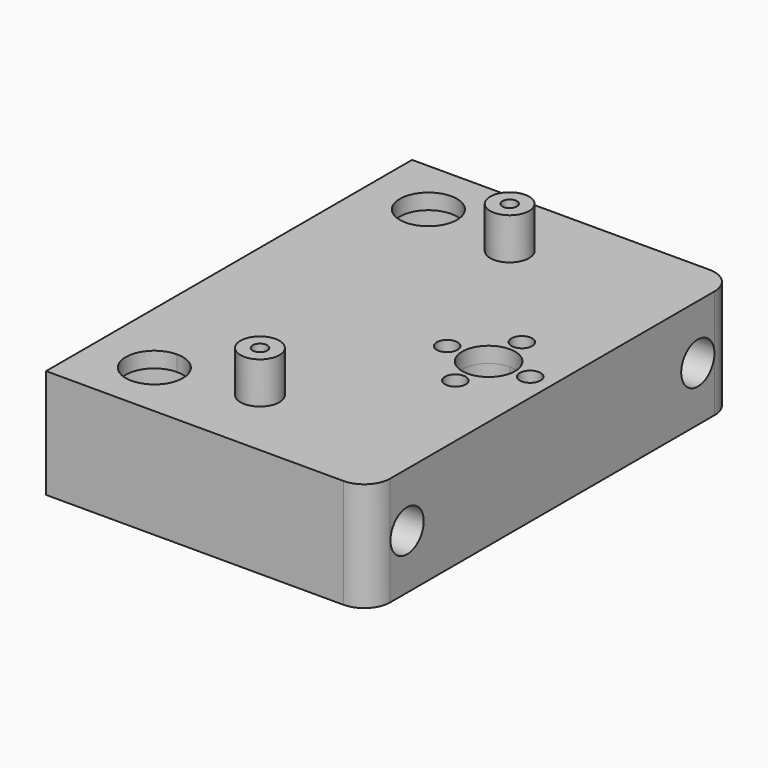
from build123d import *

# Parameters (mm, degrees)
F1_DEPTH  = 2
F2_R      = 9.75
F2_R_2    = 11.25
F2_R_3    = 2
F3_DEPTH  = 16
F4_R      = 9.75
F4_R_2    = 2
F4_R_3    = 5.1
F5_DEPTH  = 3
F7_DEPTH  = 40
F6_R      = 4
F8_DEPTH  = 35
F9_R      = 3.75
F9_R_2    = 1.4
F10_DEPTH = 8


# Not quite as in the source:
# - after a boolean that leaves OpenCascade's solid faulty, fix() repairs it
# - a feature names something its author has since deleted; it is built from what else it names


with BuildPart() as f1:
    # F0 (on Top) → F1 (new body)
    with BuildSketch(Plane.XY):
        with BuildLine():
            Line((50.2909459174, -23.5600714934), (50.2909459174, 23.5599285066))
            Line((50.2909459174, 23.5599285066), (50.2909459174, 39.0599285066))
            ThreePointArc((50.2909459174, 39.0599285066), (48.8264798233, 42.5954624125), (45.2909459174, 44.0599285066))
            Line((45.2909459174, 44.0599285066), (-12, 44.0599285066))
            Line((-12, 44.0599285066), (-12, 0))
            Line((-12, 0), (-12, -44.0599285066))
            Line((-12, -44.0599285066), (45.2909459174, -44.0599285066))
            ThreePointArc((45.2909459174, -44.0599285066), (48.8264798233, -42.5954624125), (50.2909459174, -39.0599285066))
            Line((50.2909459174, -39.0599285066), (50.2909459174, -23.5600714934))
        make_face()
        with BuildLine():
            ThreePointArc((9.75, -33), (-6.8942911166, -39.8942911166), (0, -23.25))
            ThreePointArc((0, -23.25), (6.8942911166, -26.1057088834), (9.75, -33))
        make_face(mode=Mode.SUBTRACT)
        with BuildLine():
            ThreePointArc((9.75, 33), (6.8942911166, 26.1057088834), (0, 23.25))
            ThreePointArc((0, 23.25), (-6.8942911166, 39.8942911166), (9.75, 33))
        make_face(mode=Mode.SUBTRACT)
        with BuildLine():
            ThreePointArc((26.75, 0), (38, 11.25), (49.25, 0))
            ThreePointArc((49.25, 0), (38, -11.25), (26.75, 0))
        make_face(mode=Mode.SUBTRACT)
    extrude(amount=F1_DEPTH)

    # F2 (on face) → F3 (join)
    with BuildSketch(Plane.XY.offset(2)):
        with BuildLine():
            ThreePointArc((50.2909459174, 39.0599285066), (48.8264798233, 42.5954624125), (45.2909459174, 44.0599285066))
            Line((45.2909459174, 44.0599285066), (-12, 44.0599285066))
            Line((-12, 44.0599285066), (-12, -44.0599285066))
            Line((-12, -44.0599285066), (45.2909459174, -44.0599285066))
            ThreePointArc((45.2909459174, -44.0599285066), (48.8264798233, -42.5954624125), (50.2909459174, -39.0599285066))
            Line((50.2909459174, -39.0599285066), (50.2909459174, 39.0599285066))
        make_face()
        with Locations((0, -33)):
            Circle(F2_R, mode=Mode.SUBTRACT)
        with Locations((0, 33)):
            Circle(F2_R, mode=Mode.SUBTRACT)
        with Locations((38, 0)):
            Circle(F2_R_2, mode=Mode.SUBTRACT)
        with Locations((38, 0)):
            Circle(F2_R_2)
        with Locations((38, -8)):
            Circle(F2_R_3, mode=Mode.SUBTRACT)
        with Locations((30, 0)):
            Circle(F2_R_3, mode=Mode.SUBTRACT)
        with BuildLine():
            ThreePointArc((38, 5.1), (41.6062445841, 3.6062445841), (43.1, 0))
            ThreePointArc((43.1, 0), (34.3937554159, -3.6062445841), (38, 5.1))
        make_face(mode=Mode.SUBTRACT)
        with BuildLine():
            ThreePointArc((40, 8), (39.4142135624, 6.5857864376), (38, 6))
            ThreePointArc((38, 6), (36.5857864376, 9.4142135624), (40, 8))
        make_face(mode=Mode.SUBTRACT)
        with BuildLine():
            ThreePointArc((48, 0), (46, -2), (44, 0))
            ThreePointArc((44, 0), (46, 2), (48, 0))
        make_face(mode=Mode.SUBTRACT)
    extrude(amount=F3_DEPTH)

    # F4 (on face) → F5 (join)
    with BuildSketch(Plane.XY.offset(18)):
        with BuildLine():
            Line((50.2909459174, -39.0599285066), (50.2909459174, 39.0599285066))
            ThreePointArc((50.2909459174, 39.0599285066), (48.8264798233, 42.5954624125), (45.2909459174, 44.0599285066))
            Line((45.2909459174, 44.0599285066), (-12, 44.0599285066))
            Line((-12, 44.0599285066), (-12, -44.0599285066))
            Line((-12, -44.0599285066), (45.2909459174, -44.0599285066))
            ThreePointArc((45.2909459174, -44.0599285066), (48.8264798233, -42.5954624125), (50.2909459174, -39.0599285066))
        make_face()
        with Locations((0, -33)):
            Circle(F4_R, mode=Mode.SUBTRACT)
        with Locations((38, -8)):
            Circle(F4_R_2, mode=Mode.SUBTRACT)
        with Locations((0, 33)):
            Circle(F4_R, mode=Mode.SUBTRACT)
        with Locations((30, 0)):
            Circle(F4_R_2, mode=Mode.SUBTRACT)
        with Locations((38, 0)):
            Circle(F4_R_3, mode=Mode.SUBTRACT)
        with Locations((38, 8)):
            Circle(F4_R_2, mode=Mode.SUBTRACT)
        with Locations((46, 0)):
            Circle(F4_R_2, mode=Mode.SUBTRACT)
        with Locations((0, -33)):
            Circle(F4_R)
        with Locations((0, 33)):
            Circle(F4_R)
    extrude(amount=F5_DEPTH)

    # F0 (on Top) → F7 (cut)
    with BuildSketch(Plane.XY):
        with BuildLine():
            ThreePointArc((5.5, -33), (3.8890872965, -29.1109127035), (0, -27.5))
            ThreePointArc((0, -27.5), (-3.8890872965, -36.8890872965), (5.5, -33))
        make_face()
        with BuildLine():
            ThreePointArc((5.5, 33), (-3.8890872965, 36.8890872965), (0, 27.5))
            ThreePointArc((0, 27.5), (3.8890872965, 29.1109127035), (5.5, 33))
        make_face()
    extrude(amount=F7_DEPTH, mode=Mode.SUBTRACT)

    add(f1.part.fix(), mode=Mode.REPLACE)

    # F6 (on face) → F8 (cut)
    with BuildSketch(Plane.YZ.offset(50.2909459174)):
        with Locations((35, 10.5)):
            Circle(F6_R)
        with Locations((-35, 10.5)):
            Circle(F6_R)
    extrude(amount=-F8_DEPTH, mode=Mode.SUBTRACT)

    # F9 (on face) → F10 (join)
    with BuildSketch(Plane.XY.offset(21)):
        with Locations((18, -30.0599285066)):
            Circle(F9_R)
        with Locations((18, -30.0599285066)):
            Circle(F9_R_2, mode=Mode.SUBTRACT)
        with Locations((18, 30.0599285066)):
            Circle(F9_R)
        with Locations((18, 30.0599285066)):
            Circle(F9_R_2, mode=Mode.SUBTRACT)
    extrude(amount=F10_DEPTH)


solid = f1.part
